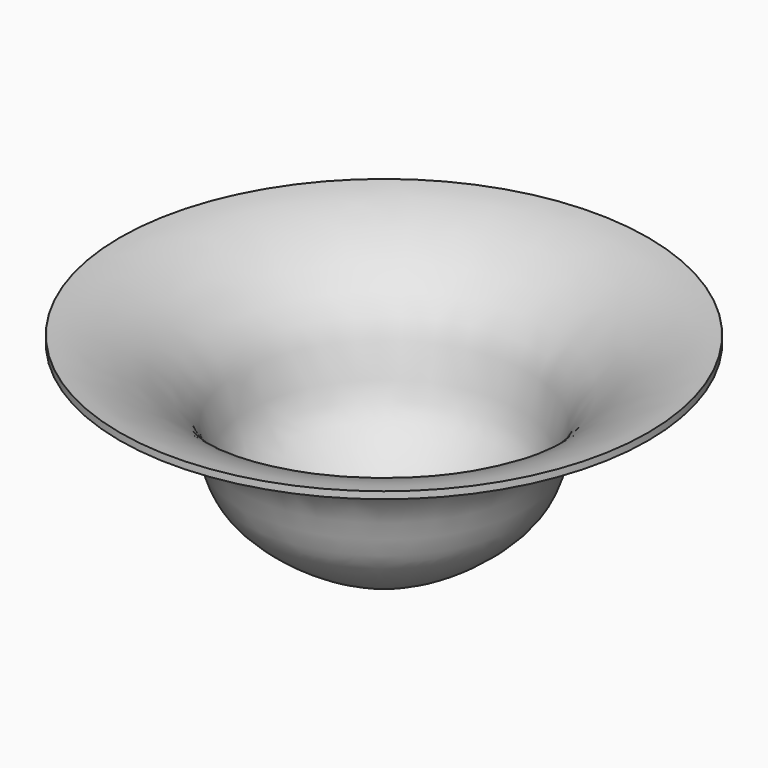
from build123d import *


# Not quite as in the source:
# - ends of sketch curves that miss each other by under 0.0002 mm in the source are joined
# - the dataset's text gives a spline's control points without its knots; the knots are read off the source's solid


with BuildPart() as f1:
    # F0 (on Front) → F1 (revolve)
    with BuildSketch(Plane.XZ):
        with BuildLine():
            Line((-7.8578934073, 0), (0, 0))
            Line((0, 0), (0, 2))
            Line((0, 2), (-7.8578934073, 2))
            Line((-7.8578934073, 2), (-7.9829875605, 2.0027392364))
            add(Edge.make_bspline(
                [(-7.9829875605, 2.0027392364), (-8.0918976762, 2.0074705535), (-8.403679734, 2.0329528901), (-9.2882877113, 2.1835728639), (-10.8673047026, 2.6236446017), (-13.1861991467, 3.5043405788), (-15.8062184782, 4.6957765634), (-18.6212240766, 6.1571538555), (-21.5333832304, 7.8475930565), (-24.4477539769, 9.7261909839), (-27.2705135228, 11.7511354585), (-29.908120585, 13.8789654513), (-32.2657522393, 16.0619538591), (-33.9202330974, 17.8838769773), (-35.0069420501, 19.305983302), (-35.9572493758, 20.7243334133), (-36.9230558568, 22.4950343504), (-37.8199969358, 24.6416191619), (-38.5393965746, 26.8298361857), (-39.3720978084, 29.817023406), (-40.1840352286, 32.91870143), (-41.3598095507, 36.1101822924), (-42.3320235989, 38.1228033268), (-43.2997624899, 39.7297828062), (-44.4061918458, 41.3226337649), (-46.0124966037, 43.248175475), (-48.2509235659, 45.4585441375), (-51.5856591491, 48.2517139142), (-56.2970861474, 51.41623485), (-62.4583252052, 54.5292420731), (-68.7724844425, 56.7741026754), (-72.8599202859, 57.5590356473), (-74.8242125434, 57.7323553895)],
                knots=[0.0045875978, 0.0045875978, 0.0045875978, 0.0045875978, 0.015625, 0.03125, 0.0625, 0.09375, 0.125, 0.15625, 0.1875, 0.21875, 0.25, 0.28125, 0.3125, 0.34375, 0.359375, 0.375, 0.40625, 0.4375, 0.46875, 0.5, 0.5625, 0.59375, 0.625, 0.640625, 0.65625, 0.6875, 0.71875, 0.75, 0.8125, 0.875, 0.9375, 1, 1, 1, 1], degree=3))
            Line((-74.8242125434, 57.7323553895), (-75, 57.7323553895))
            Line((-75, 57.7323553895), (-75, 55.740095675))
            add(Edge.make_bspline(
                [(-7.8578934073, 0), (-13.0301450225, 0), (-43.1223104294, 16.1059520109), (-39.1945312614, 40.8505202438), (-64.6183213881, 54.8240660703), (-75, 55.740095675)],
                knots=[0, 0, 0, 0, 0.3508779107, 0.6436654263, 1, 1, 1, 1], degree=3))
        make_face()
    revolve(axis=Axis((0, 0, 82.1167943617), (0, 0, 1)))


solid = f1.part
